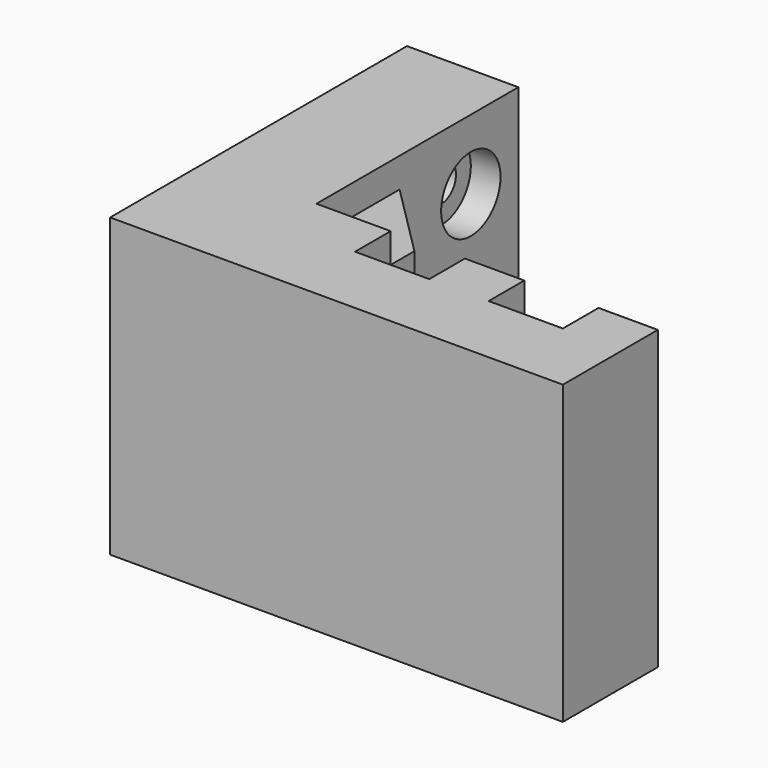
from build123d import *

# Parameters (mm, degrees)
F1_DEPTH     = 40
F2_R         = 5
F2_R_2       = 2.5
F3_DEPTH     = 4
F4_DEPTH     = 15.001
F2_W         = 14
F2_H         = 6
F5_DEPTH     = 10
F2_H_2       = 10
F6_DEPTH     = 10
F7_SIZE      = 9.99999
F8_W         = 10
F8_H         = 10
F8_W_2       = 8
F9_DEPTH     = 15
F10_T4_DEPTH = 61.4336597593


# Not quite as in the source:
# - a fillet or chamfer that OpenCascade refuses, or shapes differently, is made with other operations: its cross-section is extruded or revolved along the edge and cut away or added
# - a fillet or chamfer is up to 0.001 mm smaller than in the source, because OpenCascade refuses the exact size
# - a feature names something its author has since deleted; it is built from what else it names


with BuildPart() as f1:
    # F0 (on Top) → F1 (new body)
    with BuildSketch(Plane.XY):
        Polygon((-20.9070546148, 3.6112386312), (-20.9070546148, 37.6112386312), (-35.9070546148, 37.6112386312), (-35.9070546148, -12.3887613688), (25.0929453852, -12.3887613688), (25.0929453852, 3.6112386312), (17.0929453852, 3.6112386312), (17.0929453852, -2.3887613688), (7.0929453852, -2.3887613688), (7.0929453852, 3.6112386312), (-0.9070546148, 3.6112386312), (-0.9070546148, -2.3887613688), (-10.9070546148, -2.3887613688), (-10.9070546148, 3.6112386312), align=None)
    extrude(amount=F1_DEPTH)

    # F2 (on face) → F3 (cut)
    with BuildSketch(Plane.YZ.offset(-20.9070546148)):
        with Locations((29.6112386312, 9.4117647059)):
            Circle(F2_R)
        with Locations((29.6112386312, 9.4117647059)):
            Circle(F2_R_2, mode=Mode.SUBTRACT)
        with Locations((11.6112386312, 20)):
            Circle(F2_R)
        with Locations((11.6112386312, 20)):
            Circle(F2_R_2, mode=Mode.SUBTRACT)
        with Locations((29.6112386312, 30.5882352941)):
            Circle(F2_R)
        with Locations((29.6112386312, 30.5882352941)):
            Circle(F2_R_2, mode=Mode.SUBTRACT)
    extrude(amount=-F3_DEPTH, mode=Mode.SUBTRACT)

    # F4 (cut, through all): faces of the model
    f4_faces = [f1.faces().sort_by_distance(p)[0] for p in [
        (-20.9070546148, 29.6112386312, 9.4117647059),
        (-20.9070546148, 11.6112386312, 20),
        (-20.9070546148, 29.6112386312, 30.5882352941),
    ]]
    extrude(f4_faces, amount=-F4_DEPTH, mode=Mode.SUBTRACT)

    # F2 (on face) → F5 (join)
    with BuildSketch(Plane.YZ.offset(-20.9070546148)):
        with Locations((10.6112386312, 33)):
            Rectangle(F2_W, F2_H)
    extrude(amount=F5_DEPTH)

    # F2 (on face) → F6 (join)
    with BuildSketch(Plane.YZ.offset(-20.9070546148)):
        with Locations((10.6112386312, 5)):
            Rectangle(F2_W, F2_H_2)
    extrude(amount=F6_DEPTH)

    # F7 (size 10 in the source; OpenCascade refuses exactly that, so slightly less here)
    f7_edges = [f1.edges().sort_by_distance(p)[0] for p in [
        (-10.907055, 17.611239, 33),
    ]]
    chamfer(f7_edges, length=F7_SIZE)

    # F8 (on face) → F9 (join)
    with BuildSketch(Plane(origin=(0, -2.3887613688, 0), x_dir=(-1, 0, 0), z_dir=(0, 1, 0))):
        with Locations((-12.0929453852, 5)):
            Rectangle(F8_W, F8_H)
        with Locations((5.9070546148, 5)):
            Rectangle(F8_W, F8_H)
        with Locations((-3.0929453852, 5)):
            Rectangle(F8_W_2, F8_H)
    extrude(amount=F9_DEPTH)

    # F10: chamfer of 10 on 1 edges, made by hand


with BuildPart() as f10_tool2:
    # F10_s3 → F10_t4 (new body)
    with BuildSketch(Plane.XY.offset(-25.7168298797)):
        Polygon((-20.9070546148, 17.6112386312), (-10.9070546148, 7.6112386312), (-10.9070546148, 17.6112386312), align=None)
    extrude(amount=F10_T4_DEPTH)

    split(bisect_by=Plane.YZ.offset(-20.9070546148), keep=Keep.TOP)

    split(bisect_by=Plane.XZ.offset(-12.6112386312), keep=Keep.BOTTOM)


with BuildPart() as f1_1:
    add(f1.part)

    # F10_t1: cut F10_tool2
    add(f10_tool2.part, mode=Mode.SUBTRACT)


solid = f1_1.part
